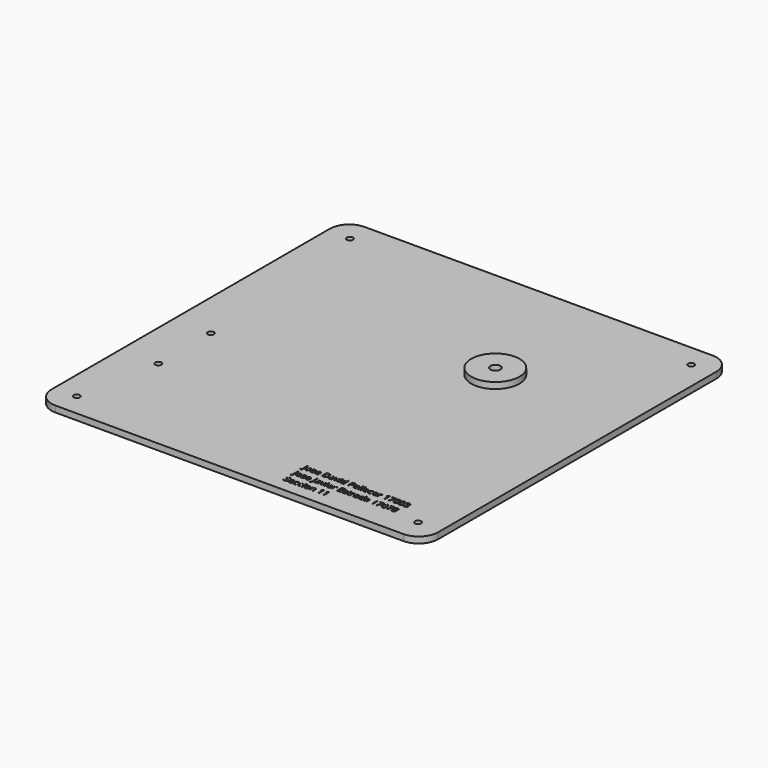
from build123d import *

# Parameters (mm, degrees)
F0_W         = 200
F0_H         = 200
F0_R         = 1.6
F0_R_2       = 2.6
F1_DEPTH     = 3.2
F2_TEXT_SIZE = 4.5989626204
F3_DEPTH     = 2.5
F4_R         = 12.5
F4_R_2       = 2.6
F5_DEPTH     = 3.2
F6_R         = 10


# Not quite as in the source:
# - Text() gives the source's letters only with a copy of the font that has no kerning and outlines rounded to 1/6400 em; it was checked with that copy


with BuildPart() as f1:
    # F0 (on Top) → F1 (new body)
    with BuildSketch(Plane.XY):
        Rectangle(F0_W, F0_H)
        with Locations((-88.2620274323, -88.2620274323)):
            Circle(F0_R, mode=Mode.SUBTRACT)
        with Locations((-80.4, -45.4)):
            Circle(F0_R, mode=Mode.SUBTRACT)
        with Locations((-80.4, -11.4)):
            Circle(F0_R, mode=Mode.SUBTRACT)
        with Locations((88.2620274323, -88.2620274323)):
            Circle(F0_R, mode=Mode.SUBTRACT)
        with Locations((-88.2620274323, 88.2620274323)):
            Circle(F0_R, mode=Mode.SUBTRACT)
        with Locations((32, 32)):
            Circle(F0_R_2, mode=Mode.SUBTRACT)
        with Locations((88.2620274323, 88.2620274323)):
            Circle(F0_R, mode=Mode.SUBTRACT)
    extrude(amount=F1_DEPTH)

    # F2 (on face) → F3 (cut)
    with BuildSketch(Plane.XY.offset(3.2)):
        with Locations((22.0695225086, -80.8967894411)):
            Text('Jose David Pellecer 17003', F2_TEXT_SIZE, font='Open Sans', text_align=(TextAlign.LEFT, TextAlign.BOTTOM))
        with Locations((22.0695225086, -87.1513786048)):
            Text('Jose Javier Estrada 17078', F2_TEXT_SIZE, font='Open Sans', text_align=(TextAlign.LEFT, TextAlign.BOTTOM))
        with Locations((22.0695225086, -93.4059677685)):
            Text('Seccion 11', F2_TEXT_SIZE, font='Open Sans', text_align=(TextAlign.LEFT, TextAlign.BOTTOM))
    extrude(amount=-F3_DEPTH, mode=Mode.SUBTRACT)

    # F6
    f6_edges = [f1.edges().sort_by_distance(p)[0] for p in [
        (100, 100, 1.6),
        (-100, 100, 1.6),
        (-100, -100, 1.6),
        (100, -100, 1.6),
    ]]
    fillet(f6_edges, radius=F6_R)


with BuildPart() as f5:
    # F4 (on face) → F5 (new body)
    with BuildSketch(Plane.XY.offset(3.2)):
        with Locations((32, 32)):
            Circle(F4_R)
        with Locations((32, 32)):
            Circle(F4_R_2, mode=Mode.SUBTRACT)
    extrude(amount=F5_DEPTH)


solid = Compound([f1.part, f5.part])
